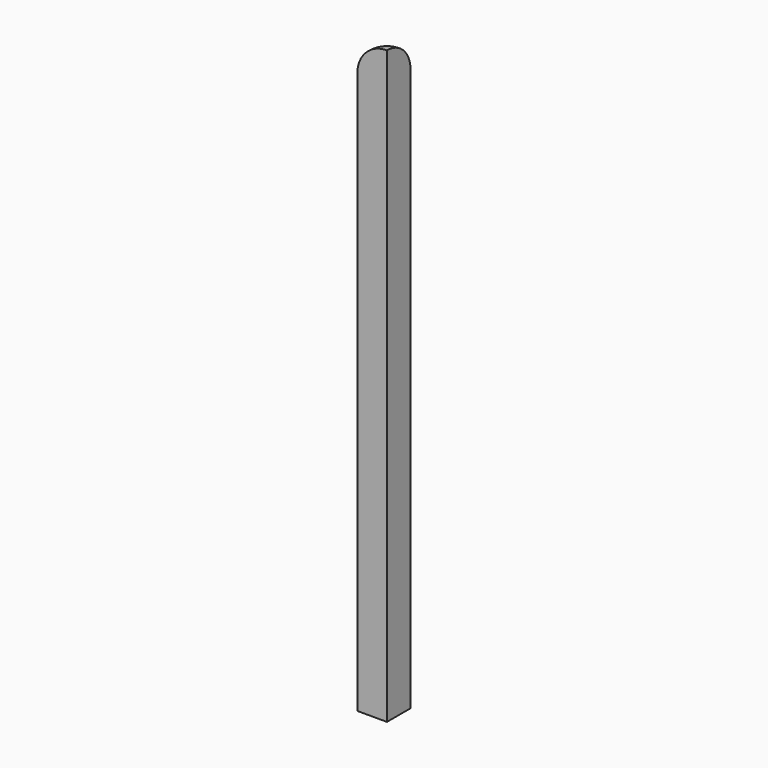
from build123d import *

# Parameters (mm, degrees)
F1_DEPTH = 100
F2_R     = 9.99999


# Not quite as in the source:
# - a fillet or chamfer is up to 0.001 mm smaller than in the source, because OpenCascade refuses the exact size


with BuildPart() as f1:
    # F0 (on Top) → F1 (new body, symmetric)
    with BuildSketch(Plane.XY):
        with BuildLine():
            Line((-5, -5), (5, -5))
            Line((5, -5), (5, 5))
            ThreePointArc((5, 5), (-2.0710678119, 2.0710678119), (-5, -5))
        make_face()
    extrude(amount=F1_DEPTH, both=True)

    # F2 (radius 10 in the source; OpenCascade refuses exactly that, so slightly less here)
    f2_edges = [f1.edges().sort_by_distance(p)[0] for p in [
        (-2.071068, 2.071068, 100),
    ]]
    fillet(f2_edges, radius=F2_R)


solid = f1.part
